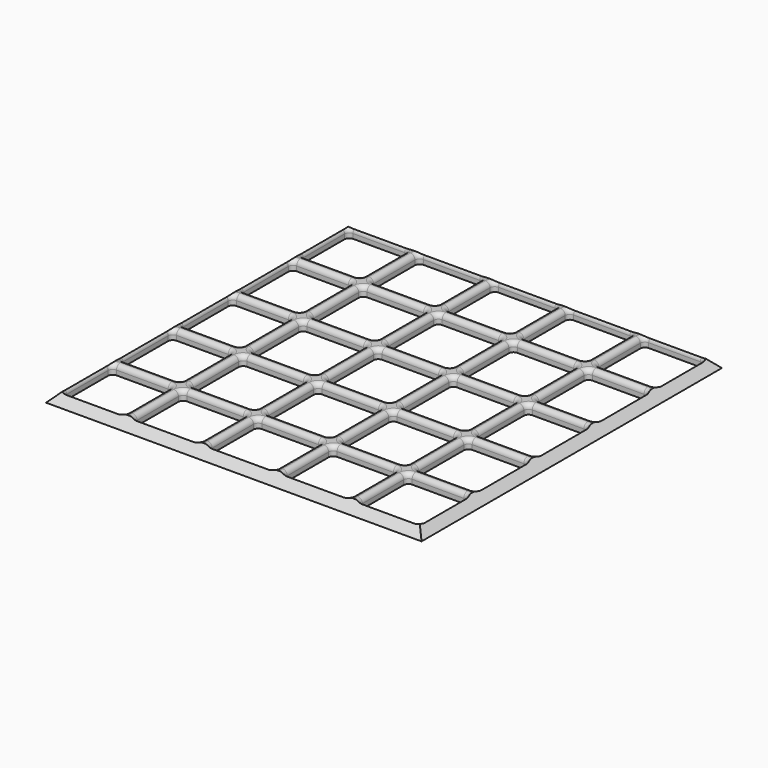
from build123d import *

# Parameters (mm, degrees)
F1_DEPTH    = 3.175
F2_R        = 1.58749
F5_T1_DEPTH = 143.3301869736
F5_T3_DEPTH = 143.3301869736


# Not quite as in the source:
# - a fillet or chamfer that OpenCascade refuses, or shapes differently, is made with other operations: its cross-section is extruded or revolved along the edge and cut away or added
# - a fillet or chamfer is up to 0.001 mm smaller than in the source, because OpenCascade refuses the exact size


with BuildPart() as f1:
    # F0 (on Top) → F1 (new body)
    with BuildSketch(Plane.XY):
        with BuildLine():
            Line((0, 63.5), (-63.5, 63.5))
            Line((-63.5, 63.5), (-63.5, 0))
            Line((-63.5, 0), (-60.325, 0))
            Line((-60.325, 0), (-60.325, 9.525))
            ThreePointArc((-60.325, 9.525), (-59.8600320151, 10.6475320151), (-58.7375, 11.1125))
            Line((-58.7375, 11.1125), (-41.275, 11.1125))
            ThreePointArc((-41.275, 11.1125), (-40.1524679849, 10.6475320151), (-39.6875, 9.525))
            Line((-39.6875, 9.525), (-39.6875, 0))
            Line((-39.6875, 0), (-36.5125, 0))
            Line((-36.5125, 0), (-36.5125, 9.525))
            ThreePointArc((-36.5125, 9.525), (-36.0475320151, 10.6475320151), (-34.925, 11.1125))
            Line((-34.925, 11.1125), (-15.875, 11.1125))
            ThreePointArc((-15.875, 11.1125), (-14.7524679849, 10.6475320151), (-14.2875, 9.525))
            Line((-14.2875, 9.525), (-14.2875, 0))
            Line((-14.2875, 0), (-11.1125, 0))
            Line((-11.1125, 0), (-11.1125, 9.525))
            ThreePointArc((-11.1125, 9.525), (-10.6475320151, 10.6475320151), (-9.525, 11.1125))
            Line((-9.525, 11.1125), (0, 11.1125))
            Line((0, 11.1125), (0, 14.2875))
            Line((0, 14.2875), (-9.525, 14.2875))
            ThreePointArc((-9.525, 14.2875), (-10.6475320151, 14.7524679849), (-11.1125, 15.875))
            Line((-11.1125, 15.875), (-11.1125, 34.925))
            ThreePointArc((-11.1125, 34.925), (-10.6475320151, 36.0475320151), (-9.525, 36.5125))
            Line((-9.525, 36.5125), (0, 36.5125))
            Line((0, 36.5125), (0, 39.6875))
            Line((0, 39.6875), (-9.525, 39.6875))
            ThreePointArc((-9.525, 39.6875), (-10.6475320151, 40.1524679849), (-11.1125, 41.275))
            Line((-11.1125, 41.275), (-11.1125, 58.7375))
            ThreePointArc((-11.1125, 58.7375), (-10.6475320151, 59.8600320151), (-9.525, 60.325))
            Line((-9.525, 60.325), (0, 60.325))
            Line((0, 60.325), (0, 63.5))
        make_face()
        with BuildLine():
            ThreePointArc((-60.325, 34.925), (-59.8600320151, 36.0475320151), (-58.7375, 36.5125))
            Line((-58.7375, 36.5125), (-41.275, 36.5125))
            ThreePointArc((-41.275, 36.5125), (-40.1524679849, 36.0475320151), (-39.6875, 34.925))
            Line((-39.6875, 34.925), (-39.6875, 15.875))
            ThreePointArc((-39.6875, 15.875), (-40.1524679849, 14.7524679849), (-41.275, 14.2875))
            Line((-41.275, 14.2875), (-58.7375, 14.2875))
            ThreePointArc((-58.7375, 14.2875), (-59.8600320151, 14.7524679849), (-60.325, 15.875))
            Line((-60.325, 15.875), (-60.325, 34.925))
        make_face(mode=Mode.SUBTRACT)
        with BuildLine():
            ThreePointArc((-36.5125, 34.925), (-36.0475320151, 36.0475320151), (-34.925, 36.5125))
            Line((-34.925, 36.5125), (-15.875, 36.5125))
            ThreePointArc((-15.875, 36.5125), (-14.7524679849, 36.0475320151), (-14.2875, 34.925))
            Line((-14.2875, 34.925), (-14.2875, 15.875))
            ThreePointArc((-14.2875, 15.875), (-14.7524679849, 14.7524679849), (-15.875, 14.2875))
            Line((-15.875, 14.2875), (-34.925, 14.2875))
            ThreePointArc((-34.925, 14.2875), (-36.0475320151, 14.7524679849), (-36.5125, 15.875))
            Line((-36.5125, 15.875), (-36.5125, 34.925))
        make_face(mode=Mode.SUBTRACT)
        with BuildLine():
            ThreePointArc((-60.325, 58.7375), (-59.8600320151, 59.8600320151), (-58.7375, 60.325))
            Line((-58.7375, 60.325), (-41.275, 60.325))
            ThreePointArc((-41.275, 60.325), (-40.1524679849, 59.8600320151), (-39.6875, 58.7375))
            Line((-39.6875, 58.7375), (-39.6875, 41.275))
            ThreePointArc((-39.6875, 41.275), (-40.1524679849, 40.1524679849), (-41.275, 39.6875))
            Line((-41.275, 39.6875), (-58.7375, 39.6875))
            ThreePointArc((-58.7375, 39.6875), (-59.8600320151, 40.1524679849), (-60.325, 41.275))
            Line((-60.325, 41.275), (-60.325, 58.7375))
        make_face(mode=Mode.SUBTRACT)
        with BuildLine():
            ThreePointArc((-36.5125, 58.7375), (-36.0475320151, 59.8600320151), (-34.925, 60.325))
            Line((-34.925, 60.325), (-15.875, 60.325))
            ThreePointArc((-15.875, 60.325), (-14.7524679849, 59.8600320151), (-14.2875, 58.7375))
            Line((-14.2875, 58.7375), (-14.2875, 41.275))
            ThreePointArc((-14.2875, 41.275), (-14.7524679849, 40.1524679849), (-15.875, 39.6875))
            Line((-15.875, 39.6875), (-34.925, 39.6875))
            ThreePointArc((-34.925, 39.6875), (-36.0475320151, 40.1524679849), (-36.5125, 41.275))
            Line((-36.5125, 41.275), (-36.5125, 58.7375))
        make_face(mode=Mode.SUBTRACT)
    extrude(amount=F1_DEPTH)

    # F2 (radius 1.5875 in the source; OpenCascade refuses exactly that, so slightly less here)
    f2_edges = [f1.edges().sort_by_distance(p)[0] for p in [
        (-60.325, 50.00625, 3.175),
        (-60.325, 25.4, 3.175),
        (-36.5125, 25.4, 3.175),
        (-36.5125, 50.00625, 3.175),
        (-11.1125, 50.00625, 3.175),
        (-11.1125, 25.4, 3.175),
        (-25.4, 11.1125, 3.175),
        (-50.00625, 11.1125, 3.175),
        (-4.7625, 11.1125, 3.175),
    ]]
    fillet(f2_edges, radius=F2_R)

    # F3: F1 across plane


with BuildPart() as f1_1:
    add(f1.part)
    add(f1.part.mirror(Plane.YZ))

    # F4: F1 across plane


with BuildPart() as f1_2:
    add(f1_1.part)
    add(f1_1.part.mirror(Plane.XZ))

    # F5: chamfer of 3.175 on 4 edges, made by hand

    # F5_s2 → F5_t1 (cut)
    with BuildSketch(Plane.YZ.offset(-71.6650934868)):
        Polygon((60.325, 3.175), (63.5, 0), (63.5, 3.175), align=None)
        Polygon((-60.325, 3.175), (-63.5, 0), (-63.5, 3.175), align=None)
    extrude(amount=F5_T1_DEPTH, mode=Mode.SUBTRACT)

    # F5_s4 → F5_t3 (cut)
    with BuildSketch(Plane.XZ.offset(-71.6650934868)):
        Polygon((-60.325, 3.175), (-63.5, 0), (-63.5, 3.175), align=None)
        Polygon((60.325, 3.175), (63.5, 0), (63.5, 3.175), align=None)
    extrude(amount=F5_T3_DEPTH, mode=Mode.SUBTRACT)


solid = f1_2.part
